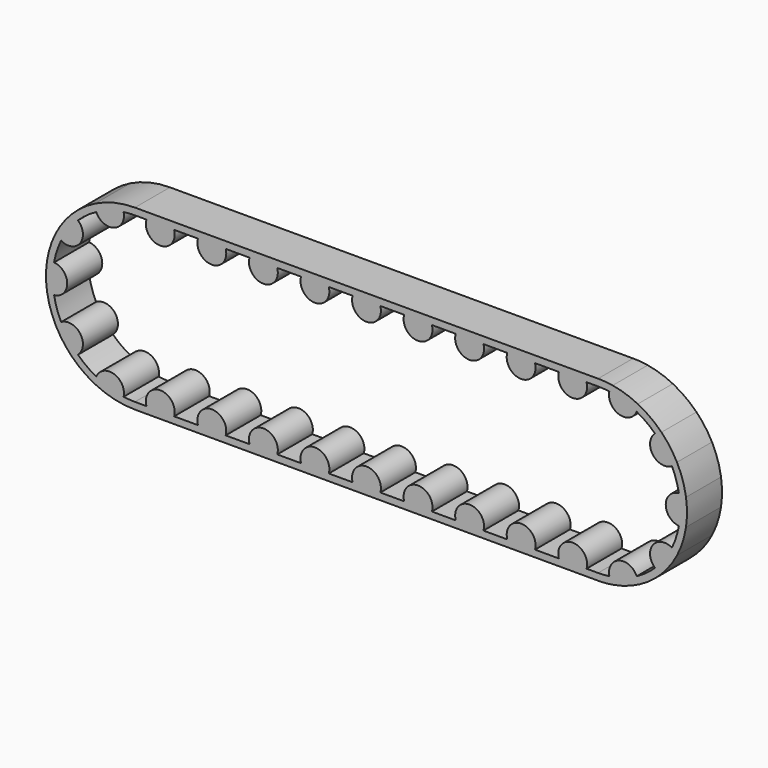
from build123d import *

# Parameters (mm, degrees)
F3_DEPTH = 25.4


with BuildPart() as f3:
    # F2 (on Front) → F3 (new body)
    with BuildSketch(Plane.XZ):
        with BuildLine():
            ThreePointArc((-6.5580901404, 47.171305671), (-3.2868824452, 47.5114410305), (0, 47.625))
            Line((0, 47.625), (6.6759446819, 47.625))
            ThreePointArc((6.6759446819, 47.625), (7.6523000339, 49.786472114), (9.1956373991, 51.5874))
            Line((9.1956373991, 51.5874), (0, 51.5874))
            ThreePointArc((0, 51.5874), (-4.2571154541, 51.4114462622), (-8.485190663, 50.8847853309))
            ThreePointArc((-8.485190663, 50.8847853309), (-7.2859359113, 49.1503637276), (-6.5580901404, 47.171305671))
        make_face()
        with BuildLine():
            ThreePointArc((-22.4209914306, 42.0171366024), (-12.129837039, 37.3317997636), (-6.5580901404, 47.171305671))
            ThreePointArc((-6.5580901404, 47.171305671), (-14.7169343571, 45.2940665886), (-22.4209914306, 42.0171366024))
        make_face()
        with BuildLine():
            ThreePointArc((-22.4209914306, 42.0171366024), (-14.7169343571, 45.2940665886), (-6.5580901404, 47.171305671))
            ThreePointArc((-6.5580901404, 47.171305671), (-7.2859359113, 49.1503637276), (-8.485190663, 50.8847853309))
            ThreePointArc((-8.485190663, 50.8847853309), (-15.9413832956, 49.0625329287), (-23.0446629367, 46.1541260224))
            ThreePointArc((-23.0446629367, 46.1541260224), (-22.9954129717, 44.0460452131), (-22.4209914306, 42.0171366024))
        make_face()
        with BuildLine():
            ThreePointArc((9.1956373991, 51.5874), (7.6523000339, 49.786472114), (6.6759446819, 47.625))
            Line((6.6759446819, 47.625), (22.7579240323, 47.625))
            ThreePointArc((22.7579240323, 47.625), (21.7815686803, 49.786472114), (20.2382313151, 51.5874))
            Line((20.2382313151, 51.5874), (9.1956373991, 51.5874))
        make_face()
        with BuildLine():
            Line((22.7579240323, 47.625), (6.6759446819, 47.625))
            ThreePointArc((6.6759446819, 47.625), (14.7169343571, 36.9220438028), (22.7579240323, 47.625))
        make_face()
        with BuildLine():
            ThreePointArc((-33.032204179, 34.307639267), (-27.9932726404, 38.5294343571), (-22.4209914306, 42.0171366024))
            ThreePointArc((-22.4209914306, 42.0171366024), (-22.9954129717, 44.0460452131), (-23.0446629367, 46.1541260224))
            ThreePointArc((-23.0446629367, 46.1541260224), (-30.3223129241, 41.7350832956), (-36.7739898304, 36.1791861533))
            ThreePointArc((-36.7739898304, 36.1791861533), (-34.7843049161, 35.4809138575), (-33.032204179, 34.307639267))
        make_face()
        with BuildLine():
            ThreePointArc((20.2382313151, 51.5874), (21.7815686803, 49.786472114), (22.7579240323, 47.625))
            Line((22.7579240323, 47.625), (36.5771902535, 47.625))
            ThreePointArc((36.5771902535, 47.625), (37.5535456055, 49.786472114), (39.0968829707, 51.5874))
            Line((39.0968829707, 51.5874), (20.2382313151, 51.5874))
        make_face()
        with BuildLine():
            ThreePointArc((-42.8360163366, 20.8138494617), (-31.7563256461, 23.0723211151), (-33.032204179, 34.307639267))
            ThreePointArc((-33.032204179, 34.307639267), (-38.5294343571, 27.9932726404), (-42.8360163366, 20.8138494617))
        make_face()
        with BuildLine():
            ThreePointArc((-42.8360163366, 20.8138494617), (-38.5294343571, 27.9932726404), (-33.032204179, 34.307639267))
            ThreePointArc((-33.032204179, 34.307639267), (-34.7843049161, 35.4809138575), (-36.7739898304, 36.1791861533))
            ThreePointArc((-36.7739898304, 36.1791861533), (-41.7350832956, 30.3223129241), (-45.7722385539, 23.7941592944))
            ThreePointArc((-45.7722385539, 23.7941592944), (-44.4932956849, 22.1176344973), (-42.8360163366, 20.8138494617))
        make_face()
        with BuildLine():
            ThreePointArc((39.0968829707, 51.5874), (37.5535456055, 49.786472114), (36.5771902535, 47.625))
            Line((36.5771902535, 47.625), (52.6591696039, 47.625))
            ThreePointArc((52.6591696039, 47.625), (51.6828142519, 49.786472114), (50.1394768867, 51.5874))
            Line((50.1394768867, 51.5874), (39.0968829707, 51.5874))
        make_face()
        with BuildLine():
            Line((52.6591696039, 47.625), (36.5771902535, 47.625))
            ThreePointArc((36.5771902535, 47.625), (44.6181799287, 36.9220438028), (52.6591696039, 47.625))
        make_face()
        with BuildLine():
            ThreePointArc((-46.8891389446, 8.3396207368), (-45.2940665886, 14.7169343571), (-42.8360163366, 20.8138494617))
            ThreePointArc((-42.8360163366, 20.8138494617), (-44.4932956849, 22.1176344973), (-45.7722385539, 23.7941592944))
            ThreePointArc((-45.7722385539, 23.7941592944), (-49.0625329287, 15.9413832956), (-51.0163747846, 7.6543675504))
            ThreePointArc((-51.0163747846, 7.6543675504), (-48.9962517179, 8.2589608458), (-46.8891389446, 8.3396207368))
        make_face()
        with BuildLine():
            ThreePointArc((50.1394768867, 51.5874), (51.6828142519, 49.786472114), (52.6591696039, 47.625))
            Line((52.6591696039, 47.625), (66.478435825, 47.625))
            ThreePointArc((66.478435825, 47.625), (67.4547911771, 49.786472114), (68.9981285423, 51.5874))
            Line((68.9981285423, 51.5874), (50.1394768867, 51.5874))
        make_face()
        with BuildLine():
            ThreePointArc((-46.8891389446, -8.3396207368), (-39.2529772142, 0), (-46.8891389446, 8.3396207368))
            ThreePointArc((-46.8891389446, 8.3396207368), (-47.625, 0), (-46.8891389446, -8.3396207368))
        make_face()
        with BuildLine():
            ThreePointArc((-46.8891389446, -8.3396207368), (-47.625, 0), (-46.8891389446, 8.3396207368))
            ThreePointArc((-46.8891389446, 8.3396207368), (-48.9962517179, 8.2589608458), (-51.0163747846, 7.6543675504))
            ThreePointArc((-51.0163747846, 7.6543675504), (-51.5874, 0), (-51.0163747846, -7.6543675504))
            ThreePointArc((-51.0163747846, -7.6543675504), (-48.9962517179, -8.2589608458), (-46.8891389446, -8.3396207368))
        make_face()
        with BuildLine():
            ThreePointArc((68.9981285423, 51.5874), (67.4547911771, 49.786472114), (66.478435825, 47.625))
            Line((66.478435825, 47.625), (82.5604151755, 47.625))
            ThreePointArc((82.5604151755, 47.625), (81.5840598235, 49.786472114), (80.0407224583, 51.5874))
            Line((80.0407224583, 51.5874), (68.9981285423, 51.5874))
        make_face()
        with BuildLine():
            Line((82.5604151755, 47.625), (66.478435825, 47.625))
            ThreePointArc((66.478435825, 47.625), (74.5194255003, 36.9220438028), (82.5604151755, 47.625))
        make_face()
        with BuildLine():
            ThreePointArc((-42.8360163366, -20.8138494617), (-45.2940665886, -14.7169343571), (-46.8891389446, -8.3396207368))
            ThreePointArc((-46.8891389446, -8.3396207368), (-48.9962517179, -8.2589608458), (-51.0163747846, -7.6543675504))
            ThreePointArc((-51.0163747846, -7.6543675504), (-49.0625329287, -15.9413832956), (-45.7722385539, -23.7941592944))
            ThreePointArc((-45.7722385539, -23.7941592944), (-44.4932956849, -22.1176344973), (-42.8360163366, -20.8138494617))
        make_face()
        with BuildLine():
            ThreePointArc((80.0407224583, 51.5874), (81.5840598235, 49.786472114), (82.5604151755, 47.625))
            Line((82.5604151755, 47.625), (96.3796813966, 47.625))
            ThreePointArc((96.3796813966, 47.625), (97.3560367487, 49.786472114), (98.8993741139, 51.5874))
            Line((98.8993741139, 51.5874), (80.0407224583, 51.5874))
        make_face()
        with BuildLine():
            ThreePointArc((-33.032204179, -34.307639267), (-31.7563256461, -23.0723211151), (-42.8360163366, -20.8138494617))
            ThreePointArc((-42.8360163366, -20.8138494617), (-38.5294343571, -27.9932726404), (-33.032204179, -34.307639267))
        make_face()
        with BuildLine():
            ThreePointArc((-33.032204179, -34.307639267), (-38.5294343571, -27.9932726404), (-42.8360163366, -20.8138494617))
            ThreePointArc((-42.8360163366, -20.8138494617), (-44.4932956849, -22.1176344973), (-45.7722385539, -23.7941592944))
            ThreePointArc((-45.7722385539, -23.7941592944), (-41.7350832956, -30.3223129241), (-36.7739898304, -36.1791861533))
            ThreePointArc((-36.7739898304, -36.1791861533), (-34.7843049161, -35.4809138575), (-33.032204179, -34.307639267))
        make_face()
        with BuildLine():
            ThreePointArc((98.8993741139, 51.5874), (97.3560367487, 49.786472114), (96.3796813966, 47.625))
            Line((96.3796813966, 47.625), (112.4616607471, 47.625))
            Line((112.4616607471, 47.625), (126.2809269682, 47.625))
            ThreePointArc((126.2809269682, 47.625), (127.2572823202, 49.786472114), (128.8006196855, 51.5874))
            Line((128.8006196855, 51.5874), (98.8993741139, 51.5874))
        make_face()
        with BuildLine():
            Line((112.4616607471, 47.625), (96.3796813966, 47.625))
            ThreePointArc((96.3796813966, 47.625), (104.4206710719, 36.9220438028), (112.4616607471, 47.625))
        make_face()
        with BuildLine():
            ThreePointArc((-22.4209914306, -42.0171366024), (-27.9932726404, -38.5294343571), (-33.032204179, -34.307639267))
            ThreePointArc((-33.032204179, -34.307639267), (-34.7843049161, -35.4809138575), (-36.7739898304, -36.1791861533))
            ThreePointArc((-36.7739898304, -36.1791861533), (-30.3223129241, -41.7350832956), (-23.0446629367, -46.1541260224))
            ThreePointArc((-23.0446629367, -46.1541260224), (-22.9954129717, -44.0460452131), (-22.4209914306, -42.0171366024))
        make_face()
        with BuildLine():
            ThreePointArc((-6.5580901404, -47.171305671), (-12.129837039, -37.3317997636), (-22.4209914306, -42.0171366024))
            ThreePointArc((-22.4209914306, -42.0171366024), (-14.7169343571, -45.2940665886), (-6.5580901404, -47.171305671))
        make_face()
        with BuildLine():
            ThreePointArc((-6.5580901404, -47.171305671), (-14.7169343571, -45.2940665886), (-22.4209914306, -42.0171366024))
            ThreePointArc((-22.4209914306, -42.0171366024), (-22.9954129717, -44.0460452131), (-23.0446629367, -46.1541260224))
            ThreePointArc((-23.0446629367, -46.1541260224), (-15.9413832956, -49.0625329287), (-8.485190663, -50.8847853309))
            ThreePointArc((-8.485190663, -50.8847853309), (-7.2859359113, -49.1503637276), (-6.5580901404, -47.171305671))
        make_face()
        with BuildLine():
            ThreePointArc((128.8006196855, 51.5874), (127.2572823202, 49.786472114), (126.2809269682, 47.625))
            Line((126.2809269682, 47.625), (142.3629063187, 47.625))
            ThreePointArc((142.3629063187, 47.625), (141.3865509666, 49.786472114), (139.8432136014, 51.5874))
            Line((139.8432136014, 51.5874), (128.8006196855, 51.5874))
        make_face()
        with BuildLine():
            Line((142.3629063187, 47.625), (126.2809269682, 47.625))
            ThreePointArc((126.2809269682, 47.625), (134.3219166434, 36.9220438028), (142.3629063187, 47.625))
        make_face()
        with BuildLine():
            ThreePointArc((0, -47.625), (-3.2868824452, -47.5114410305), (-6.5580901404, -47.171305671))
            ThreePointArc((-6.5580901404, -47.171305671), (-7.2859359113, -49.1503637276), (-8.485190663, -50.8847853309))
            ThreePointArc((-8.485190663, -50.8847853309), (-4.2571154541, -51.4114462622), (0, -51.5874))
            Line((0, -51.5874), (9.1956373991, -51.5874))
            ThreePointArc((9.1956373991, -51.5874), (7.6523000339, -49.786472114), (6.6759446819, -47.625))
            Line((6.6759446819, -47.625), (0, -47.625))
        make_face()
        with BuildLine():
            ThreePointArc((139.8432136014, 51.5874), (141.3865509666, 49.786472114), (142.3629063187, 47.625))
            Line((142.3629063187, 47.625), (156.1821725398, 47.625))
            ThreePointArc((156.1821725398, 47.625), (157.1585278918, 49.786472114), (158.701865257, 51.5874))
            Line((158.701865257, 51.5874), (139.8432136014, 51.5874))
        make_face()
        with BuildLine():
            ThreePointArc((158.701865257, 51.5874), (157.1585278918, 49.786472114), (156.1821725398, 47.625))
            Line((156.1821725398, 47.625), (172.2641518903, 47.625))
            ThreePointArc((172.2641518903, 47.625), (171.2877965382, 49.786472114), (169.744459173, 51.5874))
            Line((169.744459173, 51.5874), (158.701865257, 51.5874))
        make_face()
        with BuildLine():
            Line((172.2641518903, 47.625), (156.1821725398, 47.625))
            ThreePointArc((156.1821725398, 47.625), (164.223162215, 36.9220438028), (172.2641518903, 47.625))
        make_face()
        with BuildLine():
            ThreePointArc((22.7579240323, -47.625), (14.7169343571, -36.9220438028), (6.6759446819, -47.625))
            Line((6.6759446819, -47.625), (22.7579240323, -47.625))
        make_face()
        with BuildLine():
            Line((22.7579240323, -47.625), (6.6759446819, -47.625))
            ThreePointArc((6.6759446819, -47.625), (7.6523000339, -49.786472114), (9.1956373991, -51.5874))
            Line((9.1956373991, -51.5874), (20.2382313151, -51.5874))
            ThreePointArc((20.2382313151, -51.5874), (21.7815686803, -49.786472114), (22.7579240323, -47.625))
        make_face()
        with BuildLine():
            ThreePointArc((169.744459173, 51.5874), (171.2877965382, 49.786472114), (172.2641518903, 47.625))
            Line((172.2641518903, 47.625), (186.0834181114, 47.625))
            ThreePointArc((186.0834181114, 47.625), (187.0597734634, 49.786472114), (188.6031108286, 51.5874))
            Line((188.6031108286, 51.5874), (169.744459173, 51.5874))
        make_face()
        with BuildLine():
            Line((36.5771902535, -47.625), (22.7579240323, -47.625))
            ThreePointArc((22.7579240323, -47.625), (21.7815686803, -49.786472114), (20.2382313151, -51.5874))
            Line((20.2382313151, -51.5874), (39.0968829707, -51.5874))
            ThreePointArc((39.0968829707, -51.5874), (37.5535456055, -49.786472114), (36.5771902535, -47.625))
        make_face()
        with BuildLine():
            ThreePointArc((188.6031108286, 51.5874), (187.0597734634, 49.786472114), (186.0834181114, 47.625))
            Line((186.0834181114, 47.625), (202.1653974618, 47.625))
            ThreePointArc((202.1653974618, 47.625), (201.1890421098, 49.786472114), (199.6457047446, 51.5874))
            Line((199.6457047446, 51.5874), (188.6031108286, 51.5874))
        make_face()
        with BuildLine():
            Line((202.1653974618, 47.625), (186.0834181114, 47.625))
            ThreePointArc((186.0834181114, 47.625), (194.1244077866, 36.9220438028), (202.1653974618, 47.625))
        make_face()
        with BuildLine():
            ThreePointArc((52.6591696039, -47.625), (44.6181799287, -36.9220438028), (36.5771902535, -47.625))
            Line((36.5771902535, -47.625), (52.6591696039, -47.625))
        make_face()
        with BuildLine():
            Line((52.6591696039, -47.625), (36.5771902535, -47.625))
            ThreePointArc((36.5771902535, -47.625), (37.5535456055, -49.786472114), (39.0968829707, -51.5874))
            Line((39.0968829707, -51.5874), (50.1394768867, -51.5874))
            ThreePointArc((50.1394768867, -51.5874), (51.6828142519, -49.786472114), (52.6591696039, -47.625))
        make_face()
        with BuildLine():
            ThreePointArc((199.6457047446, 51.5874), (201.1890421098, 49.786472114), (202.1653974618, 47.625))
            Line((202.1653974618, 47.625), (215.984663683, 47.625))
            ThreePointArc((215.984663683, 47.625), (216.961019035, 49.786472114), (218.5043564002, 51.5874))
            Line((218.5043564002, 51.5874), (199.6457047446, 51.5874))
        make_face()
        with BuildLine():
            Line((66.478435825, -47.625), (52.6591696039, -47.625))
            ThreePointArc((52.6591696039, -47.625), (51.6828142519, -49.786472114), (50.1394768867, -51.5874))
            Line((50.1394768867, -51.5874), (68.9981285423, -51.5874))
            ThreePointArc((68.9981285423, -51.5874), (67.4547911771, -49.786472114), (66.478435825, -47.625))
        make_face()
        with BuildLine():
            ThreePointArc((218.5043564002, 51.5874), (216.961019035, 49.786472114), (215.984663683, 47.625))
            Line((215.984663683, 47.625), (232.0666430334, 47.625))
            ThreePointArc((232.0666430334, 47.625), (231.0902876814, 49.786472114), (229.5469503162, 51.5874))
            Line((229.5469503162, 51.5874), (218.5043564002, 51.5874))
        make_face()
        with BuildLine():
            Line((232.0666430334, 47.625), (215.984663683, 47.625))
            ThreePointArc((215.984663683, 47.625), (224.0256533582, 36.9220438028), (232.0666430334, 47.625))
        make_face()
        with BuildLine():
            ThreePointArc((82.5604151755, -47.625), (74.5194255003, -36.9220438028), (66.478435825, -47.625))
            Line((66.478435825, -47.625), (82.5604151755, -47.625))
        make_face()
        with BuildLine():
            Line((82.5604151755, -47.625), (66.478435825, -47.625))
            ThreePointArc((66.478435825, -47.625), (67.4547911771, -49.786472114), (68.9981285423, -51.5874))
            Line((68.9981285423, -51.5874), (80.0407224583, -51.5874))
            ThreePointArc((80.0407224583, -51.5874), (81.5840598235, -49.786472114), (82.5604151755, -47.625))
        make_face()
        with BuildLine():
            ThreePointArc((229.5469503162, 51.5874), (231.0902876814, 49.786472114), (232.0666430334, 47.625))
            Line((232.0666430334, 47.625), (245.8859092545, 47.625))
            ThreePointArc((245.8859092545, 47.625), (246.8622646066, 49.786472114), (248.4056019718, 51.5874))
            Line((248.4056019718, 51.5874), (229.5469503162, 51.5874))
        make_face()
        with BuildLine():
            Line((96.3796813966, -47.625), (82.5604151755, -47.625))
            ThreePointArc((82.5604151755, -47.625), (81.5840598235, -49.786472114), (80.0407224583, -51.5874))
            Line((80.0407224583, -51.5874), (98.8993741139, -51.5874))
            ThreePointArc((98.8993741139, -51.5874), (97.3560367487, -49.786472114), (96.3796813966, -47.625))
        make_face()
        with BuildLine():
            ThreePointArc((248.4056019718, 51.5874), (246.8622646066, 49.786472114), (245.8859092545, 47.625))
            Line((245.8859092545, 47.625), (261.967888605, 47.625))
            ThreePointArc((261.967888605, 47.625), (260.991533253, 49.786472114), (259.4481958878, 51.5874))
            Line((259.4481958878, 51.5874), (248.4056019718, 51.5874))
        make_face()
        with BuildLine():
            Line((261.967888605, 47.625), (245.8859092545, 47.625))
            ThreePointArc((245.8859092545, 47.625), (253.9268989298, 36.9220438028), (261.967888605, 47.625))
        make_face()
        with BuildLine():
            ThreePointArc((112.4616607471, -47.625), (104.4206710719, -36.9220438028), (96.3796813966, -47.625))
            Line((96.3796813966, -47.625), (112.4616607471, -47.625))
        make_face()
        with BuildLine():
            Line((112.4616607471, -47.625), (96.3796813966, -47.625))
            ThreePointArc((96.3796813966, -47.625), (97.3560367487, -49.786472114), (98.8993741139, -51.5874))
            Line((98.8993741139, -51.5874), (109.9419680298, -51.5874))
            ThreePointArc((109.9419680298, -51.5874), (111.485305395, -49.786472114), (112.4616607471, -47.625))
        make_face()
        with BuildLine():
            ThreePointArc((259.4481958878, 51.5874), (260.991533253, 49.786472114), (261.967888605, 47.625))
            Line((261.967888605, 47.625), (268.6438332869, 47.625))
            ThreePointArc((268.6438332869, 47.625), (271.930715732, 47.5114410305), (275.2019234272, 47.171305671))
            ThreePointArc((275.2019234272, 47.171305671), (275.9297691982, 49.1503637276), (277.1290239498, 50.8847853309))
            ThreePointArc((277.1290239498, 50.8847853309), (272.900948741, 51.4114462622), (268.6438332869, 51.5874))
            Line((268.6438332869, 51.5874), (259.4481958878, 51.5874))
        make_face()
        with BuildLine():
            Line((126.2809269682, -47.625), (112.4616607471, -47.625))
            ThreePointArc((112.4616607471, -47.625), (111.485305395, -49.786472114), (109.9419680298, -51.5874))
            Line((109.9419680298, -51.5874), (128.8006196855, -51.5874))
            ThreePointArc((128.8006196855, -51.5874), (127.2572823202, -49.786472114), (126.2809269682, -47.625))
        make_face()
        with BuildLine():
            ThreePointArc((142.3629063187, -47.625), (134.3219166434, -36.9220438028), (126.2809269682, -47.625))
            Line((126.2809269682, -47.625), (142.3629063187, -47.625))
        make_face()
        with BuildLine():
            Line((142.3629063187, -47.625), (126.2809269682, -47.625))
            ThreePointArc((126.2809269682, -47.625), (127.2572823202, -49.786472114), (128.8006196855, -51.5874))
            Line((128.8006196855, -51.5874), (139.8432136014, -51.5874))
            ThreePointArc((139.8432136014, -51.5874), (141.3865509666, -49.786472114), (142.3629063187, -47.625))
        make_face()
        with BuildLine():
            ThreePointArc((277.1290239498, 50.8847853309), (275.9297691982, 49.1503637276), (275.2019234272, 47.171305671))
            ThreePointArc((275.2019234272, 47.171305671), (283.360767644, 45.2940665886), (291.0648247175, 42.0171366024))
            ThreePointArc((291.0648247175, 42.0171366024), (291.6392462586, 44.0460452131), (291.6884962236, 46.1541260224))
            ThreePointArc((291.6884962236, 46.1541260224), (284.5852165825, 49.0625329287), (277.1290239498, 50.8847853309))
        make_face()
        with BuildLine():
            ThreePointArc((291.0648247175, 42.0171366024), (283.360767644, 45.2940665886), (275.2019234272, 47.171305671))
            ThreePointArc((275.2019234272, 47.171305671), (280.7736703259, 37.3317997636), (291.0648247175, 42.0171366024))
        make_face()
        with BuildLine():
            Line((156.1821725398, -47.625), (142.3629063187, -47.625))
            ThreePointArc((142.3629063187, -47.625), (141.3865509666, -49.786472114), (139.8432136014, -51.5874))
            Line((139.8432136014, -51.5874), (158.701865257, -51.5874))
            ThreePointArc((158.701865257, -51.5874), (157.1585278918, -49.786472114), (156.1821725398, -47.625))
        make_face()
        with BuildLine():
            ThreePointArc((291.6884962236, 46.1541260224), (291.6392462586, 44.0460452131), (291.0648247175, 42.0171366024))
            ThreePointArc((291.0648247175, 42.0171366024), (296.6371059273, 38.5294343571), (301.6760374659, 34.307639267))
            ThreePointArc((301.6760374659, 34.307639267), (303.4281382029, 35.4809138575), (305.4178231173, 36.1791861533))
            ThreePointArc((305.4178231173, 36.1791861533), (298.966146211, 41.7350832956), (291.6884962236, 46.1541260224))
        make_face()
        with BuildLine():
            ThreePointArc((172.2641518903, -47.625), (164.223162215, -36.9220438028), (156.1821725398, -47.625))
            Line((156.1821725398, -47.625), (172.2641518903, -47.625))
        make_face()
        with BuildLine():
            Line((172.2641518903, -47.625), (156.1821725398, -47.625))
            ThreePointArc((156.1821725398, -47.625), (157.1585278918, -49.786472114), (158.701865257, -51.5874))
            Line((158.701865257, -51.5874), (169.744459173, -51.5874))
            ThreePointArc((169.744459173, -51.5874), (171.2877965382, -49.786472114), (172.2641518903, -47.625))
        make_face()
        with BuildLine():
            ThreePointArc((305.4178231173, 36.1791861533), (303.4281382029, 35.4809138575), (301.6760374659, 34.307639267))
            ThreePointArc((301.6760374659, 34.307639267), (307.173267644, 27.9932726404), (311.4798496235, 20.8138494617))
            ThreePointArc((311.4798496235, 20.8138494617), (313.1371289717, 22.1176344973), (314.4160718408, 23.7941592944))
            ThreePointArc((314.4160718408, 23.7941592944), (310.3789165825, 30.3223129241), (305.4178231173, 36.1791861533))
        make_face()
        with BuildLine():
            ThreePointArc((311.4798496235, 20.8138494617), (307.173267644, 27.9932726404), (301.6760374659, 34.307639267))
            ThreePointArc((301.6760374659, 34.307639267), (300.400158933, 23.0723211151), (311.4798496235, 20.8138494617))
        make_face()
        with BuildLine():
            Line((186.0834181114, -47.625), (172.2641518903, -47.625))
            ThreePointArc((172.2641518903, -47.625), (171.2877965382, -49.786472114), (169.744459173, -51.5874))
            Line((169.744459173, -51.5874), (188.6031108286, -51.5874))
            ThreePointArc((188.6031108286, -51.5874), (187.0597734634, -49.786472114), (186.0834181114, -47.625))
        make_face()
        with BuildLine():
            ThreePointArc((314.4160718408, 23.7941592944), (313.1371289717, 22.1176344973), (311.4798496235, 20.8138494617))
            ThreePointArc((311.4798496235, 20.8138494617), (313.9378998754, 14.7169343571), (315.5329722315, 8.3396207368))
            ThreePointArc((315.5329722315, 8.3396207368), (317.6400850048, 8.2589608458), (319.6602080715, 7.6543675504))
            ThreePointArc((319.6602080715, 7.6543675504), (317.7063662156, 15.9413832956), (314.4160718408, 23.7941592944))
        make_face()
        with BuildLine():
            ThreePointArc((202.1653974618, -47.625), (194.1244077866, -36.9220438028), (186.0834181114, -47.625))
            Line((186.0834181114, -47.625), (202.1653974618, -47.625))
        make_face()
        with BuildLine():
            Line((202.1653974618, -47.625), (186.0834181114, -47.625))
            ThreePointArc((186.0834181114, -47.625), (187.0597734634, -49.786472114), (188.6031108286, -51.5874))
            Line((188.6031108286, -51.5874), (199.6457047446, -51.5874))
            ThreePointArc((199.6457047446, -51.5874), (201.1890421098, -49.786472114), (202.1653974618, -47.625))
        make_face()
        with BuildLine():
            ThreePointArc((319.6602080715, 7.6543675504), (317.6400850048, 8.2589608458), (315.5329722315, 8.3396207368))
            ThreePointArc((315.5329722315, 8.3396207368), (316.2688332869, 0), (315.5329722315, -8.3396207368))
            ThreePointArc((315.5329722315, -8.3396207368), (317.6400850048, -8.2589608458), (319.6602080715, -7.6543675504))
            ThreePointArc((319.6602080715, -7.6543675504), (320.2312332869, 0), (319.6602080715, 7.6543675504))
        make_face()
        with BuildLine():
            ThreePointArc((315.5329722315, -8.3396207368), (316.2688332869, 0), (315.5329722315, 8.3396207368))
            ThreePointArc((315.5329722315, 8.3396207368), (307.8968105011, 0), (315.5329722315, -8.3396207368))
        make_face()
        with BuildLine():
            Line((215.984663683, -47.625), (202.1653974618, -47.625))
            ThreePointArc((202.1653974618, -47.625), (201.1890421098, -49.786472114), (199.6457047446, -51.5874))
            Line((199.6457047446, -51.5874), (218.5043564002, -51.5874))
            ThreePointArc((218.5043564002, -51.5874), (216.961019035, -49.786472114), (215.984663683, -47.625))
        make_face()
        with BuildLine():
            ThreePointArc((319.6602080715, -7.6543675504), (317.6400850048, -8.2589608458), (315.5329722315, -8.3396207368))
            ThreePointArc((315.5329722315, -8.3396207368), (313.9378998754, -14.7169343571), (311.4798496235, -20.8138494617))
            ThreePointArc((311.4798496235, -20.8138494617), (313.1371289717, -22.1176344973), (314.4160718408, -23.7941592944))
            ThreePointArc((314.4160718408, -23.7941592944), (317.7063662156, -15.9413832956), (319.6602080715, -7.6543675504))
        make_face()
        with BuildLine():
            ThreePointArc((232.0666430334, -47.625), (224.0256533582, -36.9220438028), (215.984663683, -47.625))
            Line((215.984663683, -47.625), (232.0666430334, -47.625))
        make_face()
        with BuildLine():
            Line((232.0666430334, -47.625), (215.984663683, -47.625))
            ThreePointArc((215.984663683, -47.625), (216.961019035, -49.786472114), (218.5043564002, -51.5874))
            Line((218.5043564002, -51.5874), (229.5469503162, -51.5874))
            ThreePointArc((229.5469503162, -51.5874), (231.0902876814, -49.786472114), (232.0666430334, -47.625))
        make_face()
        with BuildLine():
            ThreePointArc((314.4160718408, -23.7941592944), (313.1371289717, -22.1176344973), (311.4798496235, -20.8138494617))
            ThreePointArc((311.4798496235, -20.8138494617), (307.173267644, -27.9932726404), (301.6760374659, -34.307639267))
            ThreePointArc((301.6760374659, -34.307639267), (303.4281382029, -35.4809138575), (305.4178231173, -36.1791861533))
            ThreePointArc((305.4178231173, -36.1791861533), (310.3789165825, -30.3223129241), (314.4160718408, -23.7941592944))
        make_face()
        with BuildLine():
            ThreePointArc((301.6760374659, -34.307639267), (307.173267644, -27.9932726404), (311.4798496235, -20.8138494617))
            ThreePointArc((311.4798496235, -20.8138494617), (300.400158933, -23.0723211151), (301.6760374659, -34.307639267))
        make_face()
        with BuildLine():
            Line((245.8859092545, -47.625), (232.0666430334, -47.625))
            ThreePointArc((232.0666430334, -47.625), (231.0902876814, -49.786472114), (229.5469503162, -51.5874))
            Line((229.5469503162, -51.5874), (248.4056019718, -51.5874))
            ThreePointArc((248.4056019718, -51.5874), (246.8622646066, -49.786472114), (245.8859092545, -47.625))
        make_face()
        with BuildLine():
            ThreePointArc((305.4178231173, -36.1791861533), (303.4281382029, -35.4809138575), (301.6760374659, -34.307639267))
            ThreePointArc((301.6760374659, -34.307639267), (296.6371059273, -38.5294343571), (291.0648247175, -42.0171366024))
            ThreePointArc((291.0648247175, -42.0171366024), (283.360767644, -45.2940665886), (275.2019234272, -47.171305671))
            ThreePointArc((275.2019234272, -47.171305671), (275.9297691982, -49.1503637276), (277.1290239498, -50.8847853309))
            ThreePointArc((277.1290239498, -50.8847853309), (292.4379925813, -45.7722385539), (305.4178231173, -36.1791861533))
        make_face()
        with BuildLine():
            ThreePointArc((261.967888605, -47.625), (253.9268989298, -36.9220438028), (245.8859092545, -47.625))
            Line((245.8859092545, -47.625), (261.967888605, -47.625))
        make_face()
        with BuildLine():
            Line((261.967888605, -47.625), (245.8859092545, -47.625))
            ThreePointArc((245.8859092545, -47.625), (246.8622646066, -49.786472114), (248.4056019718, -51.5874))
            Line((248.4056019718, -51.5874), (259.4481958878, -51.5874))
            ThreePointArc((259.4481958878, -51.5874), (260.991533253, -49.786472114), (261.967888605, -47.625))
        make_face()
        with BuildLine():
            ThreePointArc((275.2019234272, -47.171305671), (283.360767644, -45.2940665886), (291.0648247175, -42.0171366024))
            ThreePointArc((291.0648247175, -42.0171366024), (280.7736703259, -37.3317997636), (275.2019234272, -47.171305671))
        make_face()
        with BuildLine():
            ThreePointArc((268.6438332869, -51.5874), (272.900948741, -51.4114462622), (277.1290239498, -50.8847853309))
            ThreePointArc((277.1290239498, -50.8847853309), (275.9297691982, -49.1503637276), (275.2019234272, -47.171305671))
            ThreePointArc((275.2019234272, -47.171305671), (271.930715732, -47.5114410305), (268.6438332869, -47.625))
            Line((268.6438332869, -47.625), (261.967888605, -47.625))
            ThreePointArc((261.967888605, -47.625), (260.991533253, -49.786472114), (259.4481958878, -51.5874))
            Line((259.4481958878, -51.5874), (268.6438332869, -51.5874))
        make_face()
    extrude(amount=F3_DEPTH)


solid = f3.part
